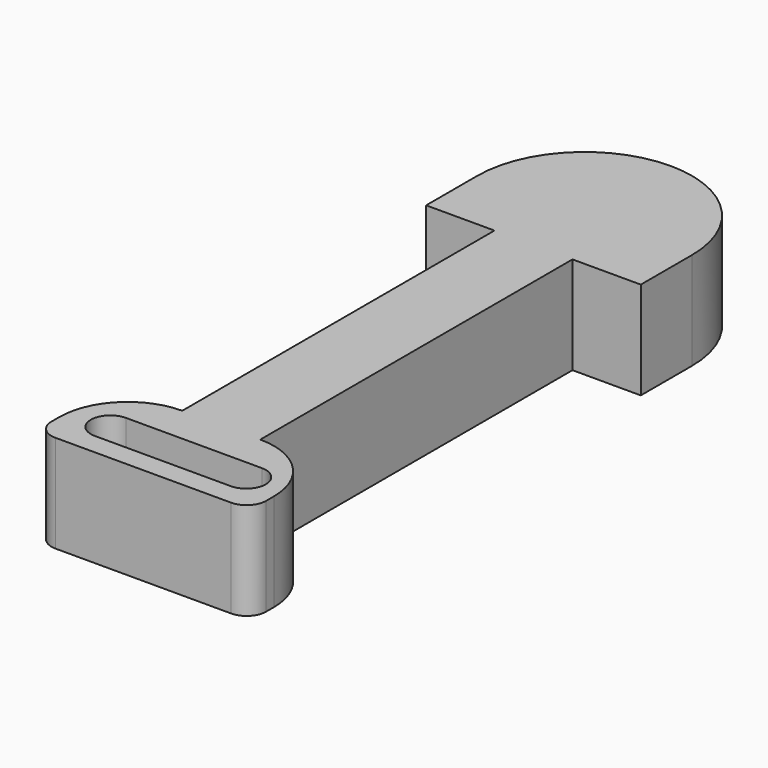
from build123d import *

# Parameters (mm, degrees)
F0_W     = 101.6
F0_H     = 508
F1_DEPTH = 127
F2_R     = 88.89999
F3_R     = 88.89999
F5_DEPTH = 127.001
F6_R     = 25.4
F7_R     = 25.4


# Not quite as in the source:
# - a fillet or chamfer is up to 0.001 mm smaller than in the source, because OpenCascade refuses the exact size


with BuildPart() as f1:
    # F0 (on Top) → F1 (new body)
    with BuildSketch(Plane.XY):
        with BuildLine():
            ThreePointArc((139.7, 83.3142390684), (0, 223.0142390684), (-139.7, 83.3142390684))
            Line((-139.7, 83.3142390684), (-139.7, 0))
            Line((-139.7, 0), (-50.8, 0))
            Line((-50.8, 0), (50.8, 0))
            Line((50.8, 0), (139.7, 0))
            Line((139.7, 0), (139.7, 83.3142390684))
        make_face()
        with Locations((0, -254)):
            Rectangle(F0_W, F0_H)
        Polygon((50.8, -508), (-50.8, -508), (-139.7, -508), (-139.7, -635), (139.7, -635), (139.7, -508), align=None)
    extrude(amount=F1_DEPTH)

    # F2 (radius 88.9 in the source; OpenCascade refuses exactly that, so slightly less here)
    f2_edges = [f1.edges().sort_by_distance(p)[0] for p in [
        (139.7, -508, 63.5),
    ]]
    fillet(f2_edges, radius=F2_R)

    # F3 (radius 88.9 in the source; OpenCascade refuses exactly that, so slightly less here)
    f3_edges = [f1.edges().sort_by_distance(p)[0] for p in [
        (-139.7, -508, 63.5),
    ]]
    fillet(f3_edges, radius=F3_R)

    # F4 (on face) → F5 (cut, through all)
    with BuildSketch(Plane.XY.offset(127)):
        with BuildLine():
            Line((91.3110496293, -556.0355413279), (-85.6204037596, -556.0355413279))
            ThreePointArc((-85.6204037596, -556.0355413279), (-111.0204037596, -581.4355413279), (-85.6204037596, -606.8355413279))
            Line((-85.6204037596, -606.8355413279), (91.3110496293, -606.8355413279))
            ThreePointArc((91.3110496293, -606.8355413279), (116.7110496293, -581.4355413279), (91.3110496293, -556.0355413279))
        make_face()
    extrude(amount=-F5_DEPTH, mode=Mode.SUBTRACT)

    # F6
    f6_edges = [f1.edges().sort_by_distance(p)[0] for p in [
        (139.7, -635, 63.5),
    ]]
    fillet(f6_edges, radius=F6_R)

    # F7
    f7_edges = [f1.edges().sort_by_distance(p)[0] for p in [
        (-139.7, -635, 63.5),
    ]]
    fillet(f7_edges, radius=F7_R)


solid = f1.part
